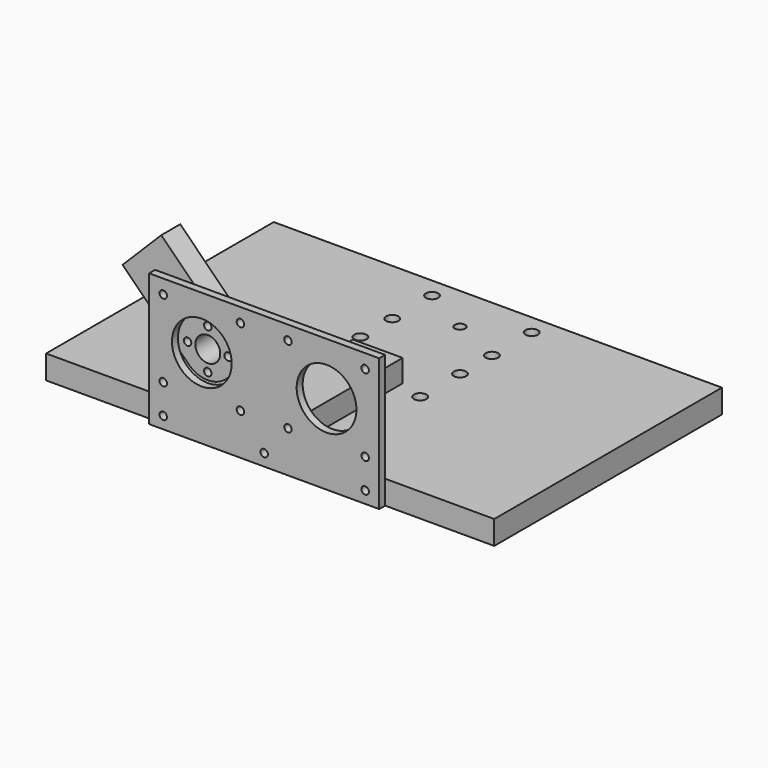
from build123d import *

# Parameters (mm, degrees)
F0_W      = 20
F0_H      = 9
F1_DEPTH  = 54
F0_W_2    = 180
F0_H_2    = 5.5153320081
F2_DEPTH  = 114.3
F3_R      = 2.5
F3_R_2    = 2.1
F4_DEPTH  = 25
F6_R      = 1.5
F6_R_2    = 5
F7_DEPTH  = 9.525
F5_W      = 42.3
F5_H      = 42.3
F5_R      = 1.5
F5_R_2    = 12
F5_W_2    = 7.8
F8_DEPTH  = 3
F9_DEPTH  = 10
F10_R     = 2.5
F11_DEPTH = 9
F13_R     = 1.1
F14_DEPTH = 25


# Not quite as in the source:
# - a feature names something its author has since deleted; it is built from what else it names


with BuildPart() as f1:
    # F0 (on Front) → F1 (new body)
    with BuildSketch(Plane.XZ):
        with Locations((0, 8.5096679919)):
            Rectangle(F0_W, F0_H)
    extrude(amount=-F1_DEPTH)

    # F10 (on face) → F11 (cut, through all)
    with BuildSketch(Plane.XY.offset(13.0096679919)):
        with Locations((0, 44)):
            Circle(F10_R)
        with Locations((0, 10)):
            Circle(F10_R)
    extrude(amount=-F11_DEPTH, mode=Mode.SUBTRACT)


with BuildPart() as f2:
    # F0 (on Front) → F2 (new body)
    with BuildSketch(Plane.XZ):
        with Locations((0, -2.7576660041)):
            Rectangle(F0_W_2, F0_H_2)
        Polygon((-90, 4.0096679919), (-90, 0), (90, 0), (90, 4.0096679919), (10, 4.0096679919), (-10, 4.0096679919), align=None)
    extrude(amount=-F2_DEPTH)

    # F3 (on face) → F4 (cut)
    with BuildSketch(Plane.XY.offset(13.0096679919)):
        with Locations((-20, 50.3)):
            Circle(F3_R)
        with Locations((20, 50.3)):
            Circle(F3_R)
        with Locations((-20, 70.3)):
            Circle(F3_R)
        with Locations((-20, 86.3)):
            Circle(F3_R)
        with Locations((-20, 106.3)):
            Circle(F3_R)
        with Locations((20, 106.3)):
            Circle(F3_R)
        with Locations((20, 86.3)):
            Circle(F3_R)
        with Locations((20, 70.3)):
            Circle(F3_R)
        with Locations((-40, 25.15)):
            Circle(F3_R)
        with Locations((0, 95.3)):
            Circle(F3_R_2)
        with Locations((0, 61.3)):
            Circle(F3_R_2)
    extrude(amount=-F4_DEPTH, mode=Mode.SUBTRACT)

    # F5 (on Front) → F9 (cut)
    with BuildSketch(Plane.XZ):
        with Locations((-40.55, -0.7528320081)):
            Circle(F5_R)
        with Locations((0, -0.7528320081)):
            Circle(F5_R)
        with Locations((40.55, -0.7528320081)):
            Circle(F5_R)
    extrude(amount=-F9_DEPTH, mode=Mode.SUBTRACT)


with BuildPart() as f7:
    # F6 (on Front) → F7 (new body)
    with BuildSketch(Plane.XZ):
        with BuildLine():
            ThreePointArc((-36.2193395846, 22.2726583904), (-33.5352813742, 35.1449493661), (-20.6629903985, 37.8290075765))
            Line((-20.6629903985, 37.8290075765), (-43.7251262658, 60.8911434438))
            Line((-43.7251262658, 60.8911434438), (-59.281475452, 45.3347942577))
            Line((-59.281475452, 45.3347942577), (-36.2193395846, 22.2726583904))
        make_face()
        with BuildLine():
            Line((-17.2718254069, 34.4378425849), (-20.6629903985, 37.8290075765))
            ThreePointArc((-20.6629903985, 37.8290075765), (-33.5352813742, 35.1449493661), (-36.2193395846, 22.2726583904))
            Line((-36.2193395846, 22.2726583904), (-32.8281745931, 18.8814933988))
            ThreePointArc((-32.8281745931, 18.8814933988), (-32.8281745931, 34.4378425849), (-17.2718254069, 34.4378425849))
        make_face()
        with BuildLine():
            ThreePointArc((-14.05, 26.6596679919), (-14.8873251424, 30.8691857479), (-17.2718254069, 34.4378425849))
            ThreePointArc((-17.2718254069, 34.4378425849), (-32.8281745931, 34.4378425849), (-32.8281745931, 18.8814933988))
            ThreePointArc((-32.8281745931, 18.8814933988), (-20.840482244, 16.4969931343), (-14.05, 26.6596679919))
        make_face()
        with Locations((-25.05, 18.5279400082)):
            Circle(F6_R, mode=Mode.SUBTRACT)
        with Locations((-33.1817279836, 26.6596679919)):
            Circle(F6_R, mode=Mode.SUBTRACT)
        with Locations((-25.05, 26.6596679919)):
            Circle(F6_R_2, mode=Mode.SUBTRACT)
        with Locations((-25.05, 34.7913959755)):
            Circle(F6_R, mode=Mode.SUBTRACT)
        with Locations((-16.9182720164, 26.6596679919)):
            Circle(F6_R, mode=Mode.SUBTRACT)
    extrude(amount=-F7_DEPTH)

    # F13 (on face) → F14 (cut)
    with BuildSketch(Plane(origin=(-52.3081348548, 0, 52.3081348548), x_dir=(0, -1, 0), z_dir=(-0.7071067812, 0, 0.7071067812))):
        with Locations((-4.525, -5.8617928475)):
            Circle(F13_R)
        with Locations((-4.525, 8.1382071525)):
            Circle(F13_R)
    extrude(amount=-F14_DEPTH, mode=Mode.SUBTRACT)


with BuildPart() as f8:
    # F5 (on Front) → F8 (new body)
    with BuildSketch(Plane.XZ):
        with Locations((-25.05, 26.6596679919)):
            Rectangle(F5_W, F5_H)
        with Locations((-40.55, 11.1596679919)):
            Circle(F5_R, mode=Mode.SUBTRACT)
        with Locations((-9.55, 11.1596679919)):
            Circle(F5_R, mode=Mode.SUBTRACT)
        with Locations((-25.05, 26.6596679919)):
            Circle(F5_R_2, mode=Mode.SUBTRACT)
        with Locations((-40.55, 42.1596679919)):
            Circle(F5_R, mode=Mode.SUBTRACT)
        with Locations((-9.55, 42.1596679919)):
            Circle(F5_R, mode=Mode.SUBTRACT)
        Polygon((46.2, 47.8096679919), (3.9, 47.8096679919), (3.9, 5.5096679919), (10, 5.5096679919), (46.2, 5.5096679919), align=None)
        with BuildLine():
            ThreePointArc((11.05, 11.1596679919), (10.7593386622, 10.2722560244), (10, 9.7287591898))
            ThreePointArc((10, 9.7287591898), (8.05, 11.1596679919), (10, 12.590576794))
            ThreePointArc((10, 12.590576794), (10.7593386622, 12.0470799593), (11.05, 11.1596679919))
        make_face(mode=Mode.SUBTRACT)
        with Locations((40.55, 11.1596679919)):
            Circle(F5_R, mode=Mode.SUBTRACT)
        with Locations((25.05, 26.6596679919)):
            Circle(F5_R_2, mode=Mode.SUBTRACT)
        with Locations((9.55, 42.1596679919)):
            Circle(F5_R, mode=Mode.SUBTRACT)
        with Locations((40.55, 42.1596679919)):
            Circle(F5_R, mode=Mode.SUBTRACT)
        with Locations((0, 26.6596679919)):
            Rectangle(F5_W_2, F5_H)
        Polygon((3.9, 5.5096679919), (-3.9, 5.5096679919), (-46.2, 5.5096679919), (-46.2, -5.5153320081), (46.2, -5.5153320081), (46.2, 5.5096679919), (10, 5.5096679919), align=None)
        with Locations((-40.55, -0.7528320081)):
            Circle(F5_R, mode=Mode.SUBTRACT)
        with Locations((0, -0.7528320081)):
            Circle(F5_R, mode=Mode.SUBTRACT)
        with Locations((40.55, -0.7528320081)):
            Circle(F5_R, mode=Mode.SUBTRACT)
    extrude(amount=F8_DEPTH)


solid = Compound([f1.part, f2.part, f7.part, f8.part])
